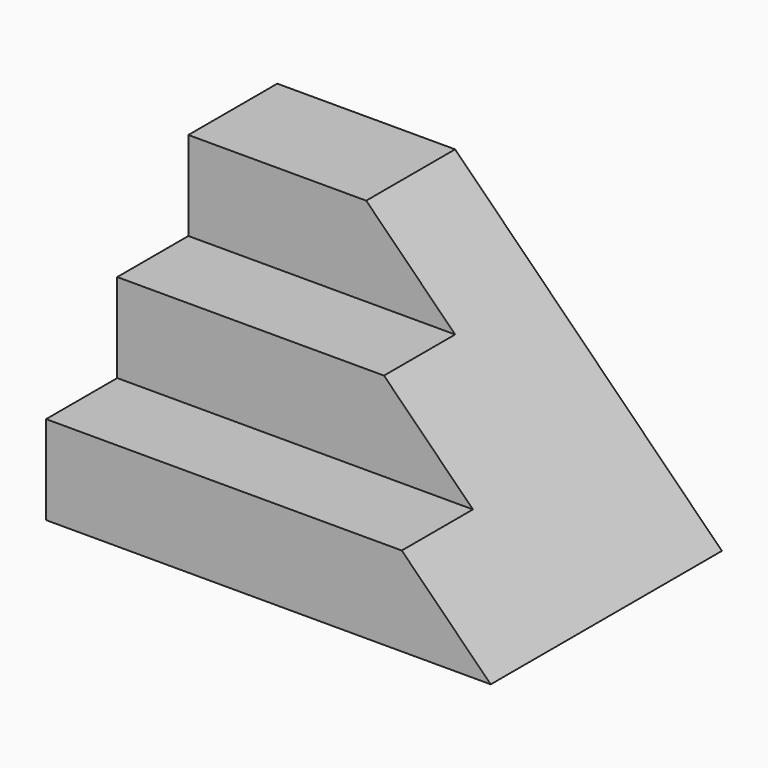
from build123d import *

# Parameters (mm, degrees)
F0_W     = 100
F0_H     = 20
F1_DEPTH = 25
F2_DEPTH = 20
F3_DEPTH = 40
F4_SIZE  = 59.99999


# Not quite as in the source:
# - a fillet or chamfer is up to 0.001 mm smaller than in the source, because OpenCascade refuses the exact size


with BuildPart() as f1:
    # F0 (on Front) → F1 (new body)
    with BuildSketch(Plane.XZ):
        with Locations((50, 10)):
            Rectangle(F0_W, F0_H)
        with Locations((50, 30)):
            Rectangle(F0_W, F0_H)
        with Locations((50, 50)):
            Rectangle(F0_W, F0_H)
    extrude(amount=-F1_DEPTH)

    # F0 (on Front) → F2 (join)
    with BuildSketch(Plane.XZ):
        with Locations((50, 30)):
            Rectangle(F0_W, F0_H)
        with Locations((50, 10)):
            Rectangle(F0_W, F0_H)
    extrude(amount=F2_DEPTH)

    # F0 (on Front) → F3 (join)
    with BuildSketch(Plane.XZ):
        with Locations((50, 10)):
            Rectangle(F0_W, F0_H)
    extrude(amount=F3_DEPTH)

    # F4 (size 60 in the source; OpenCascade refuses exactly that, so slightly less here)
    f4_edges = [f1.edges().sort_by_distance(p)[0] for p in [
        (100, 12.5, 60),
    ]]
    chamfer(f4_edges, length=F4_SIZE)


solid = f1.part
